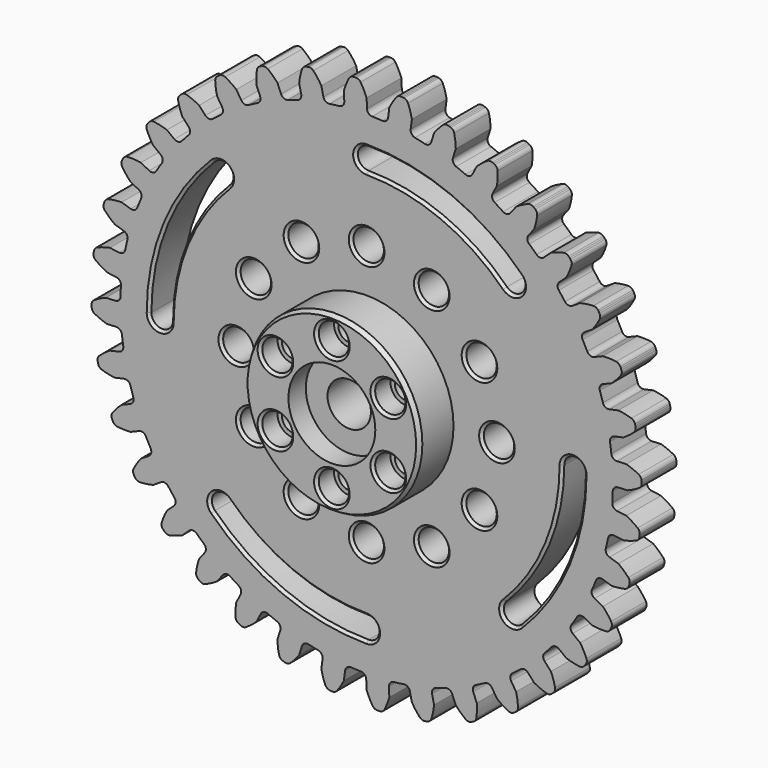
from build123d import *

# Parameters (mm, degrees)
F1_DEPTH       = 6.35
F2_R           = 2.2225
F3_DEPTH       = 25.4
F4_R           = 12.7
F5_DEPTH       = 6.35
F7_D           = 3.175
F7_CBORE_D     = 4.445
F7_CBORE_DEPTH = 3.175
F8_D           = 6.35
F8_CBORE_D     = 12.7
F8_CBORE_DEPTH = 3.175
F9_SIZE2       = 0.6599113577
F9_SIZE        = 0.381
F10_SIZE2      = 0.381
F10_SIZE       = 0.381


with BuildPart() as f1:
    # F0 (on Front) → F1 (new body)
    with BuildSketch(Plane.XZ):
        with BuildLine():
            ThreePointArc((-3.2606716013, 36.5816578877), (-3.4493856486, 36.0349930627), (-3.9606537478, 35.7646962753))
            ThreePointArc((-3.9606537478, 35.7646962753), (-4.6967674834, 35.6754909284), (-5.4308867943, 35.5711364227))
            ThreePointArc((-5.4308867943, 35.5711364227), (-5.9946918119, 35.6998971492), (-6.318462852, 36.1790920324))
            Line((-6.318462852, 36.1790920324), (-6.6159955691, 37.5211753898))
            ThreePointArc((-6.6159955691, 37.5211753898), (-7.1619458758, 38.3313229182), (-7.7880082615, 39.081287347))
            ThreePointArc((-7.7880082615, 39.081287347), (-8.1146145803, 39.2926127714), (-8.5025305694, 39.3217899538))
            Line((-8.5025305694, 39.3217899538), (-8.7093463733, 39.2853227475))
            Line((-8.7093463733, 39.2853227475), (-8.9121968543, 39.2309691249))
            ThreePointArc((-8.9121968543, 39.2309691249), (-9.2514373257, 39.0405852364), (-9.4581331923, 38.7110295639))
            ThreePointArc((-9.4581331923, 38.7110295639), (-9.7085897444, 37.7667455649), (-9.8610056184, 36.8017739816))
            Line((-9.8610056184, 36.8017739816), (-9.5634729013, 35.4596906243))
            ThreePointArc((-9.5634729013, 35.4596906243), (-9.6543926075, 34.8885610159), (-10.1109568509, 34.5335898704))
            ThreePointArc((-10.1109568509, 34.5335898704), (-10.8203970188, 34.3179149444), (-11.5252424382, 34.0876673376))
            ThreePointArc((-11.5252424382, 34.0876673376), (-12.1028410562, 34.1165681854), (-12.5049046048, 34.5322607706))
            Line((-12.5049046048, 34.5322607706), (-13.0309674607, 35.8022888519))
            ThreePointArc((-13.0309674607, 35.8022888519), (-13.7093041974, 36.5053251432), (-14.4560852451, 37.1351813348))
            ThreePointArc((-14.4560852451, 37.1351813348), (-14.8144259549, 37.286581659), (-15.201515193, 37.2479546698))
            Line((-15.201515193, 37.2479546698), (-15.3988565363, 37.1761282949))
            Line((-15.3988565363, 37.1761282949), (-15.5891868551, 37.0873758097))
            ThreePointArc((-15.5891868551, 37.0873758097), (-15.8902136862, 36.8409757905), (-16.0365426362, 36.4805344486))
            ThreePointArc((-16.0365426362, 36.4805344486), (-16.1192209948, 35.5071049215), (-16.1017557723, 34.5303266861))
            Line((-16.1017557723, 34.5303266861), (-15.5756929164, 33.2602986047))
            ThreePointArc((-15.5756929164, 33.2602986047), (-15.5660557323, 32.6820576972), (-15.9540436464, 32.2531978121))
            ThreePointArc((-15.9540436464, 32.2531978121), (-16.6152542662, 31.9176064805), (-17.2694094225, 31.5684617296))
            ThreePointArc((-17.2694094225, 31.5684617296), (-17.8432515992, 31.4966245612), (-18.311391159, 31.8361842394))
            Line((-18.311391159, 31.8361842394), (-19.05, 32.9955678842))
            ThreePointArc((-19.05, 32.9955678842), (-19.8401122483, 33.5701315363), (-20.6849213937, 34.060741629))
            ThreePointArc((-20.6849213937, 34.060741629), (-21.0641084934, 34.1476166309), (-21.4386094698, 34.0423591317))
            Line((-21.4386094698, 34.0423591317), (-21.6204802356, 33.9373559961))
            Line((-21.6204802356, 33.9373559961), (-21.7925073018, 33.8169013475))
            ThreePointArc((-21.7925073018, 33.8169013475), (-22.0461739447, 33.5219719377), (-22.127689847, 33.1415967542))
            ThreePointArc((-22.127689847, 33.1415967542), (-22.0400778721, 32.1685988626), (-21.853262225, 31.2096928874))
            Line((-21.853262225, 31.2096928874), (-21.114653384, 30.0503092426))
            ThreePointArc((-21.114653384, 30.0503092426), (-21.0047521305, 29.4825265932), (-21.3123748989, 28.9928086592))
            ThreePointArc((-21.3123748989, 28.9928086592), (-21.9052654205, 28.5474976948), (-22.4888541403, 28.0900643864))
            ThreePointArc((-22.4888541403, 28.0900643864), (-23.0415039716, 27.9196719377), (-23.5614953589, 28.17278136))
            Line((-23.5614953589, 28.17278136), (-24.4902079291, 29.1862932828))
            ThreePointArc((-24.4902079291, 29.1862932828), (-25.3680885281, 29.61492647), (-26.2852566728, 29.9513835244))
            ThreePointArc((-26.2852566728, 29.9513835244), (-26.6737687542, 29.9710935509), (-27.0243024464, 29.8024037375))
            Line((-27.0243024464, 29.8024037375), (-27.1851765834, 29.6674143085))
            Line((-27.1851765834, 29.6674143085), (-27.3336734418, 29.5189174501))
            ThreePointArc((-27.3336734418, 29.5189174501), (-27.5322723638, 29.1844199304), (-27.5464983989, 28.7956684128))
            ThreePointArc((-27.5464983989, 28.7956684128), (-27.291258136, 27.8526662053), (-26.9407683632, 26.9407683632))
            Line((-26.9407683632, 26.9407683632), (-26.012055793, 25.9272564403))
            ThreePointArc((-26.012055793, 25.9272564403), (-25.8052297641, 25.3871838375), (-26.0231404246, 24.8514876862))
            ThreePointArc((-26.0231404246, 24.8514876862), (-26.5296961696, 24.3099876374), (-27.024986405, 23.758164651))
            ThreePointArc((-27.024986405, 23.758164651), (-27.5396519053, 23.4943942104), (-28.095695445, 23.653362775))
            Line((-28.095695445, 23.653362775), (-29.1862932828, 24.4902079291))
            ThreePointArc((-29.1862932828, 24.4902079291), (-30.1252682748, 24.7598868487), (-31.0869277289, 24.9319677875))
            ThreePointArc((-31.0869277289, 24.9319677875), (-31.472960049, 24.8839139595), (-31.7888756681, 24.6569173866))
            Line((-31.7888756681, 24.6569173866), (-31.9238650971, 24.4960432496))
            Line((-31.9238650971, 24.4960432496), (-32.0443197457, 24.3240161833))
            ThreePointArc((-32.0443197457, 24.3240161833), (-32.1818166191, 23.9601140917), (-32.1283205362, 23.5747982581))
            ThreePointArc((-32.1283205362, 23.5747982581), (-31.7132073315, 22.6904443795), (-31.2096928874, 21.853262225))
            Line((-31.2096928874, 21.853262225), (-30.1190950495, 21.0164170709))
            ThreePointArc((-30.1190950495, 21.0164170709), (-29.8216285495, 20.5204643475), (-29.9432059969, 19.9550668353))
            ThreePointArc((-29.9432059969, 19.9550668353), (-30.3480355252, 19.333830907), (-30.7399781331, 18.704385105))
            ThreePointArc((-30.7399781331, 18.704385105), (-31.2010214516, 18.3552512038), (-31.7762220421, 18.4152487314))
            Line((-31.7762220421, 18.4152487314), (-32.9955678842, 19.05))
            ThreePointArc((-32.9955678842, 19.05), (-33.9671069891, 19.1525305947), (-34.9440382167, 19.1550068256))
            ThreePointArc((-34.9440382167, 19.1550068256), (-35.3158613788, 19.0406492343), (-35.5875599885, 18.7622430779))
            Line((-35.5875599885, 18.7622430779), (-35.6925631241, 18.5803723121))
            Line((-35.6925631241, 18.5803723121), (-35.7813156093, 18.3900419933))
            ThreePointArc((-35.7813156093, 18.3900419933), (-35.8535326612, 18.0077923106), (-35.7339399116, 17.6376197876))
            ThreePointArc((-35.7339399116, 17.6376197876), (-35.1715667699, 16.8387848831), (-34.5303266861, 16.1017557723))
            Line((-34.5303266861, 16.1017557723), (-33.310980844, 15.4670045037))
            ThreePointArc((-33.310980844, 15.4670045037), (-32.9319122418, 15.0302409322), (-32.953462407, 14.4523213765))
            ThreePointArc((-32.953462407, 14.4523213765), (-33.2442651782, 13.7702255079), (-33.5209511807, 13.0822822824))
            ThreePointArc((-33.5209511807, 13.0822822824), (-33.9143637496, 12.6583931776), (-34.4912442119, 12.6175966735))
            Line((-34.4912442119, 12.6175966735), (-35.8022888519, 13.0309674607))
            ThreePointArc((-35.8022888519, 13.0309674607), (-36.7768723457, 12.9632343902), (-37.7393917859, 12.7960306742))
            ThreePointArc((-37.7393917859, 12.7960306742), (-38.0857081313, 12.6188440172), (-38.3049343069, 12.2974875074))
            Line((-38.3049343069, 12.2974875074), (-38.3767606818, 12.1001461641))
            Line((-38.3767606818, 12.1001461641), (-38.4311143044, 11.8972956831))
            ThreePointArc((-38.4311143044, 11.8972956831), (-38.4358572562, 11.5083128726), (-38.2538016052, 11.164531165))
            ThreePointArc((-38.2538016052, 11.164531165), (-37.5612559497, 10.4754874289), (-36.8017739816, 9.8610056184))
            Line((-36.8017739816, 9.8610056184), (-35.4907293416, 9.4476348312))
            ThreePointArc((-35.4907293416, 9.4476348312), (-35.041576445, 9.0833312518), (-34.9624445371, 8.5104494458))
            ThreePointArc((-34.9624445371, 8.5104494458), (-35.1303846562, 7.7882187749), (-35.2834070892, 7.0626809326))
            ThreePointArc((-35.2834070892, 7.0626809326), (-35.5972352666, 6.5769162801), (-36.1582673798, 6.4365653256))
            Line((-36.1582673798, 6.4365653256), (-37.5211753898, 6.6159955691))
            ThreePointArc((-37.5211753898, 6.6159955691), (-38.4691910462, 6.3800568684), (-39.3880530326, 6.0482536059))
            ThreePointArc((-39.3880530326, 6.0482536059), (-39.6983399145, 5.81362161), (-39.8584325796, 5.4590790018))
            Line((-39.8584325796, 5.4590790018), (-39.8948997859, 5.2522631978))
            Line((-39.8948997859, 5.2522631978), (-39.9132030384, 5.043056064))
            ThreePointArc((-39.9132030384, 5.043056064), (-39.8503277779, 4.6591591714), (-39.6113408943, 4.3522139125))
            ThreePointArc((-39.6113408943, 4.3522139125), (-38.8096653743, 3.79389759), (-37.9550179973, 3.3206337987))
            Line((-37.9550179973, 3.3206337987), (-36.5921099874, 3.1412035552))
            ThreePointArc((-36.5921099874, 3.1412035552), (-36.0865200798, 2.8604291477), (-35.9091104818, 2.3099918152))
            ThreePointArc((-35.9091104818, 2.3099918152), (-35.9490851733, 1.5695709554), (-35.9737945275, 0.8284835965))
            ThreePointArc((-35.9737945275, 0.8284835965), (-36.198502803, 0.2956031095), (-36.7266398904, 0.0599621973))
            Line((-36.7266398904, 0.0599621973), (-38.1, 0))
            ThreePointArc((-38.1, 0), (-38.992642843, -0.3969754528), (-39.8399282193, -0.8832965877))
            ThreePointArc((-39.8399282193, -0.8832965877), (-40.1047577277, -1.1682447479), (-40.2008525477, -1.5452008569))
            Line((-40.2008525477, -1.5452008569), (-40.2008525477, -1.755207128))
            Line((-40.2008525477, -1.755207128), (-40.1825492952, -1.9644142618))
            ThreePointArc((-40.1825492952, -1.9644142618), (-40.0539662553, -2.3315607235), (-39.7653096346, -2.5923431574))
            ThreePointArc((-39.7653096346, -2.5923431574), (-38.8788627552, -3.0029679073), (-37.9550179973, -3.3206337987))
            Line((-37.9550179973, -3.3206337987), (-36.5816578877, -3.2606716013))
            ThreePointArc((-36.5816578877, -3.2606716013), (-36.0349930627, -3.4493856486), (-35.7646962753, -3.9606537478))
            ThreePointArc((-35.7646962753, -3.9606537478), (-35.6754909284, -4.6967674834), (-35.5711364227, -5.4308867943))
            ThreePointArc((-35.5711364227, -5.4308867943), (-35.6998971492, -5.9946918119), (-36.1790920324, -6.318462852))
            Line((-36.1790920324, -6.318462852), (-37.5211753898, -6.6159955691))
            ThreePointArc((-37.5211753898, -6.6159955691), (-38.3313229182, -7.1619458758), (-39.081287347, -7.7880082615))
            ThreePointArc((-39.081287347, -7.7880082615), (-39.2926127714, -8.1146145803), (-39.3217899538, -8.5025305694))
            Line((-39.3217899538, -8.5025305694), (-39.2853227475, -8.7093463733))
            Line((-39.2853227475, -8.7093463733), (-39.2309691249, -8.9121968543))
            ThreePointArc((-39.2309691249, -8.9121968543), (-39.0405852364, -9.2514373257), (-38.7110295639, -9.4581331923))
            ThreePointArc((-38.7110295639, -9.4581331923), (-37.7667455649, -9.7085897444), (-36.8017739816, -9.8610056184))
            Line((-36.8017739816, -9.8610056184), (-35.4596906243, -9.5634729013))
            ThreePointArc((-35.4596906243, -9.5634729013), (-34.8885610159, -9.6543926075), (-34.5335898704, -10.1109568509))
            ThreePointArc((-34.5335898704, -10.1109568509), (-34.3179149444, -10.8203970188), (-34.0876673376, -11.5252424382))
            ThreePointArc((-34.0876673376, -11.5252424382), (-34.1165681854, -12.1028410562), (-34.5322607706, -12.5049046048))
            Line((-34.5322607706, -12.5049046048), (-35.8022888519, -13.0309674607))
            ThreePointArc((-35.8022888519, -13.0309674607), (-36.5053251432, -13.7093041974), (-37.1351813348, -14.4560852451))
            ThreePointArc((-37.1351813348, -14.4560852451), (-37.286581659, -14.8144259549), (-37.2479546698, -15.201515193))
            Line((-37.2479546698, -15.201515193), (-37.1761282949, -15.3988565363))
            Line((-37.1761282949, -15.3988565363), (-37.0873758097, -15.5891868551))
            ThreePointArc((-37.0873758097, -15.5891868551), (-36.8409757905, -15.8902136862), (-36.4805344486, -16.0365426362))
            ThreePointArc((-36.4805344486, -16.0365426362), (-35.5071049215, -16.1192209948), (-34.5303266861, -16.1017557723))
            Line((-34.5303266861, -16.1017557723), (-33.2602986047, -15.5756929164))
            ThreePointArc((-33.2602986047, -15.5756929164), (-32.6820576972, -15.5660557323), (-32.2531978121, -15.9540436464))
            ThreePointArc((-32.2531978121, -15.9540436464), (-31.9176064805, -16.6152542662), (-31.5684617296, -17.2694094225))
            ThreePointArc((-31.5684617296, -17.2694094225), (-31.4966245612, -17.8432515992), (-31.8361842394, -18.311391159))
            Line((-31.8361842394, -18.311391159), (-32.9955678842, -19.05))
            ThreePointArc((-32.9955678842, -19.05), (-33.5701315363, -19.8401122483), (-34.060741629, -20.6849213937))
            ThreePointArc((-34.060741629, -20.6849213937), (-34.1476166309, -21.0641084934), (-34.0423591317, -21.4386094698))
            Line((-34.0423591317, -21.4386094698), (-33.9373559961, -21.6204802356))
            Line((-33.9373559961, -21.6204802356), (-33.8169013475, -21.7925073018))
            ThreePointArc((-33.8169013475, -21.7925073018), (-33.5219719377, -22.0461739447), (-33.1415967542, -22.127689847))
            ThreePointArc((-33.1415967542, -22.127689847), (-32.1685988626, -22.0400778721), (-31.2096928874, -21.853262225))
            Line((-31.2096928874, -21.853262225), (-30.0503092426, -21.114653384))
            ThreePointArc((-30.0503092426, -21.114653384), (-29.4825265932, -21.0047521305), (-28.9928086592, -21.3123748989))
            ThreePointArc((-28.9928086592, -21.3123748989), (-28.5474976948, -21.9052654205), (-28.0900643864, -22.4888541403))
            ThreePointArc((-28.0900643864, -22.4888541403), (-27.9196719377, -23.0415039716), (-28.17278136, -23.5614953589))
            Line((-28.17278136, -23.5614953589), (-29.1862932828, -24.4902079291))
            ThreePointArc((-29.1862932828, -24.4902079291), (-29.61492647, -25.3680885281), (-29.9513835244, -26.2852566728))
            ThreePointArc((-29.9513835244, -26.2852566728), (-29.9710935509, -26.6737687542), (-29.8024037375, -27.0243024464))
            Line((-29.8024037375, -27.0243024464), (-29.6674143085, -27.1851765834))
            Line((-29.6674143085, -27.1851765834), (-29.5189174501, -27.3336734418))
            ThreePointArc((-29.5189174501, -27.3336734418), (-29.1844199304, -27.5322723638), (-28.7956684128, -27.5464983989))
            ThreePointArc((-28.7956684128, -27.5464983989), (-27.8526662053, -27.291258136), (-26.9407683632, -26.9407683632))
            Line((-26.9407683632, -26.9407683632), (-25.9272564403, -26.012055793))
            ThreePointArc((-25.9272564403, -26.012055793), (-25.3871838375, -25.8052297641), (-24.8514876862, -26.0231404246))
            ThreePointArc((-24.8514876862, -26.0231404246), (-24.3099876374, -26.5296961696), (-23.758164651, -27.024986405))
            ThreePointArc((-23.758164651, -27.024986405), (-23.4943942104, -27.5396519053), (-23.653362775, -28.095695445))
            Line((-23.653362775, -28.095695445), (-24.4902079291, -29.1862932828))
            ThreePointArc((-24.4902079291, -29.1862932828), (-24.7598868487, -30.1252682748), (-24.9319677875, -31.0869277289))
            ThreePointArc((-24.9319677875, -31.0869277289), (-24.8839139595, -31.472960049), (-24.6569173866, -31.7888756681))
            Line((-24.6569173866, -31.7888756681), (-24.4960432496, -31.9238650971))
            Line((-24.4960432496, -31.9238650971), (-24.3240161833, -32.0443197457))
            ThreePointArc((-24.3240161833, -32.0443197457), (-23.9601140917, -32.1818166191), (-23.5747982581, -32.1283205362))
            ThreePointArc((-23.5747982581, -32.1283205362), (-22.6904443795, -31.7132073315), (-21.853262225, -31.2096928874))
            Line((-21.853262225, -31.2096928874), (-21.0164170709, -30.1190950495))
            ThreePointArc((-21.0164170709, -30.1190950495), (-20.5204643475, -29.8216285495), (-19.9550668353, -29.9432059969))
            ThreePointArc((-19.9550668353, -29.9432059969), (-19.333830907, -30.3480355252), (-18.704385105, -30.7399781331))
            ThreePointArc((-18.704385105, -30.7399781331), (-18.3552512038, -31.2010214516), (-18.4152487314, -31.7762220421))
            Line((-18.4152487314, -31.7762220421), (-19.05, -32.9955678842))
            ThreePointArc((-19.05, -32.9955678842), (-19.1525305947, -33.9671069891), (-19.1550068256, -34.9440382167))
            ThreePointArc((-19.1550068256, -34.9440382167), (-19.0406492343, -35.3158613788), (-18.7622430779, -35.5875599885))
            Line((-18.7622430779, -35.5875599885), (-18.5803723121, -35.6925631241))
            Line((-18.5803723121, -35.6925631241), (-18.3900419933, -35.7813156093))
            ThreePointArc((-18.3900419933, -35.7813156093), (-18.0077923106, -35.8535326612), (-17.6376197876, -35.7339399116))
            ThreePointArc((-17.6376197876, -35.7339399116), (-16.8387848831, -35.1715667699), (-16.1017557723, -34.5303266861))
            Line((-16.1017557723, -34.5303266861), (-15.4670045037, -33.310980844))
            ThreePointArc((-15.4670045037, -33.310980844), (-15.0302409322, -32.9319122418), (-14.4523213765, -32.953462407))
            ThreePointArc((-14.4523213765, -32.953462407), (-13.7702255079, -33.2442651782), (-13.0822822824, -33.5209511807))
            ThreePointArc((-13.0822822824, -33.5209511807), (-12.6583931776, -33.9143637496), (-12.6175966735, -34.4912442119))
            Line((-12.6175966735, -34.4912442119), (-13.0309674607, -35.8022888519))
            ThreePointArc((-13.0309674607, -35.8022888519), (-12.9632343902, -36.7768723457), (-12.7960306742, -37.7393917859))
            ThreePointArc((-12.7960306742, -37.7393917859), (-12.6188440172, -38.0857081313), (-12.2974875074, -38.3049343069))
            Line((-12.2974875074, -38.3049343069), (-12.1001461641, -38.3767606818))
            Line((-12.1001461641, -38.3767606818), (-11.8972956831, -38.4311143044))
            ThreePointArc((-11.8972956831, -38.4311143044), (-11.5083128726, -38.4358572562), (-11.164531165, -38.2538016052))
            ThreePointArc((-11.164531165, -38.2538016052), (-10.4754874289, -37.5612559497), (-9.8610056184, -36.8017739816))
            Line((-9.8610056184, -36.8017739816), (-9.4476348312, -35.4907293416))
            ThreePointArc((-9.4476348312, -35.4907293416), (-9.0833312518, -35.041576445), (-8.5104494458, -34.9624445371))
            ThreePointArc((-8.5104494458, -34.9624445371), (-7.7882187749, -35.1303846562), (-7.0626809326, -35.2834070892))
            ThreePointArc((-7.0626809326, -35.2834070892), (-6.5769162801, -35.5972352666), (-6.4365653256, -36.1582673798))
            Line((-6.4365653256, -36.1582673798), (-6.6159955691, -37.5211753898))
            ThreePointArc((-6.6159955691, -37.5211753898), (-6.3800568684, -38.4691910462), (-6.0482536059, -39.3880530326))
            ThreePointArc((-6.0482536059, -39.3880530326), (-5.81362161, -39.6983399145), (-5.4590790018, -39.8584325796))
            Line((-5.4590790018, -39.8584325796), (-5.2522631978, -39.8948997859))
            Line((-5.2522631978, -39.8948997859), (-5.043056064, -39.9132030384))
            ThreePointArc((-5.043056064, -39.9132030384), (-4.6591591714, -39.8503277779), (-4.3522139125, -39.6113408943))
            ThreePointArc((-4.3522139125, -39.6113408943), (-3.79389759, -38.8096653743), (-3.3206337987, -37.9550179973))
            Line((-3.3206337987, -37.9550179973), (-3.1412035552, -36.5921099874))
            ThreePointArc((-3.1412035552, -36.5921099874), (-2.8604291477, -36.0865200798), (-2.3099918152, -35.9091104818))
            ThreePointArc((-2.3099918152, -35.9091104818), (-1.5695709554, -35.9490851733), (-0.8284835965, -35.9737945275))
            ThreePointArc((-0.8284835965, -35.9737945275), (-0.2956031095, -36.198502803), (-0.0599621973, -36.7266398904))
            Line((-0.0599621973, -36.7266398904), (0, -38.1))
            ThreePointArc((0, -38.1), (0.3969754528, -38.992642843), (0.8832965877, -39.8399282193))
            ThreePointArc((0.8832965877, -39.8399282193), (1.1682447479, -40.1047577277), (1.5452008569, -40.2008525477))
            Line((1.5452008569, -40.2008525477), (1.755207128, -40.2008525477))
            Line((1.755207128, -40.2008525477), (1.9644142618, -40.1825492952))
            ThreePointArc((1.9644142618, -40.1825492952), (2.3315607235, -40.0539662553), (2.5923431574, -39.7653096346))
            ThreePointArc((2.5923431574, -39.7653096346), (3.0029679073, -38.8788627552), (3.3206337987, -37.9550179973))
            Line((3.3206337987, -37.9550179973), (3.2606716013, -36.5816578877))
            ThreePointArc((3.2606716013, -36.5816578877), (3.4493856486, -36.0349930627), (3.9606537478, -35.7646962753))
            ThreePointArc((3.9606537478, -35.7646962753), (4.6967674834, -35.6754909284), (5.4308867943, -35.5711364227))
            ThreePointArc((5.4308867943, -35.5711364227), (5.9946918119, -35.6998971492), (6.318462852, -36.1790920324))
            Line((6.318462852, -36.1790920324), (6.6159955691, -37.5211753898))
            ThreePointArc((6.6159955691, -37.5211753898), (7.1619458758, -38.3313229182), (7.7880082615, -39.081287347))
            ThreePointArc((7.7880082615, -39.081287347), (8.1146145803, -39.2926127714), (8.5025305694, -39.3217899538))
            Line((8.5025305694, -39.3217899538), (8.7093463733, -39.2853227475))
            Line((8.7093463733, -39.2853227475), (8.9121968543, -39.2309691249))
            ThreePointArc((8.9121968543, -39.2309691249), (9.2514373257, -39.0405852364), (9.4581331923, -38.7110295639))
            ThreePointArc((9.4581331923, -38.7110295639), (9.7085897444, -37.7667455649), (9.8610056184, -36.8017739816))
            Line((9.8610056184, -36.8017739816), (9.5634729013, -35.4596906243))
            ThreePointArc((9.5634729013, -35.4596906243), (9.6543926075, -34.8885610159), (10.1109568509, -34.5335898704))
            ThreePointArc((10.1109568509, -34.5335898704), (10.8203970188, -34.3179149444), (11.5252424382, -34.0876673376))
            ThreePointArc((11.5252424382, -34.0876673376), (12.1028410562, -34.1165681854), (12.5049046048, -34.5322607706))
            Line((12.5049046048, -34.5322607706), (13.0309674607, -35.8022888519))
            ThreePointArc((13.0309674607, -35.8022888519), (13.7093041974, -36.5053251432), (14.4560852451, -37.1351813348))
            ThreePointArc((14.4560852451, -37.1351813348), (14.8144259549, -37.286581659), (15.201515193, -37.2479546698))
            Line((15.201515193, -37.2479546698), (15.3988565363, -37.1761282949))
            Line((15.3988565363, -37.1761282949), (15.5891868551, -37.0873758097))
            ThreePointArc((15.5891868551, -37.0873758097), (15.8902136862, -36.8409757905), (16.0365426362, -36.4805344486))
            ThreePointArc((16.0365426362, -36.4805344486), (16.1192209948, -35.5071049215), (16.1017557723, -34.5303266861))
            Line((16.1017557723, -34.5303266861), (15.5756929164, -33.2602986047))
            ThreePointArc((15.5756929164, -33.2602986047), (15.5660557323, -32.6820576972), (15.9540436464, -32.2531978121))
            ThreePointArc((15.9540436464, -32.2531978121), (16.6152542662, -31.9176064805), (17.2694094225, -31.5684617296))
            ThreePointArc((17.2694094225, -31.5684617296), (17.8432515992, -31.4966245612), (18.311391159, -31.8361842394))
            Line((18.311391159, -31.8361842394), (19.05, -32.9955678842))
            ThreePointArc((19.05, -32.9955678842), (19.8401122483, -33.5701315363), (20.6849213937, -34.060741629))
            ThreePointArc((20.6849213937, -34.060741629), (21.0641084934, -34.1476166309), (21.4386094698, -34.0423591317))
            Line((21.4386094698, -34.0423591317), (21.6204802356, -33.9373559961))
            Line((21.6204802356, -33.9373559961), (21.7925073018, -33.8169013475))
            ThreePointArc((21.7925073018, -33.8169013475), (22.0461739447, -33.5219719377), (22.127689847, -33.1415967542))
            ThreePointArc((22.127689847, -33.1415967542), (22.0400778721, -32.1685988626), (21.853262225, -31.2096928874))
            Line((21.853262225, -31.2096928874), (21.114653384, -30.0503092426))
            ThreePointArc((21.114653384, -30.0503092426), (21.0047521305, -29.4825265932), (21.3123748989, -28.9928086592))
            ThreePointArc((21.3123748989, -28.9928086592), (21.9052654205, -28.5474976948), (22.4888541403, -28.0900643864))
            ThreePointArc((22.4888541403, -28.0900643864), (23.0415039716, -27.9196719377), (23.5614953589, -28.17278136))
            Line((23.5614953589, -28.17278136), (24.4902079291, -29.1862932828))
            ThreePointArc((24.4902079291, -29.1862932828), (25.3680885281, -29.61492647), (26.2852566728, -29.9513835244))
            ThreePointArc((26.2852566728, -29.9513835244), (26.6737687542, -29.9710935509), (27.0243024464, -29.8024037375))
            Line((27.0243024464, -29.8024037375), (27.1851765834, -29.6674143085))
            Line((27.1851765834, -29.6674143085), (27.3336734418, -29.5189174501))
            ThreePointArc((27.3336734418, -29.5189174501), (27.5322723638, -29.1844199304), (27.5464983989, -28.7956684128))
            ThreePointArc((27.5464983989, -28.7956684128), (27.291258136, -27.8526662053), (26.9407683632, -26.9407683632))
            Line((26.9407683632, -26.9407683632), (26.012055793, -25.9272564403))
            ThreePointArc((26.012055793, -25.9272564403), (25.8052297641, -25.3871838375), (26.0231404246, -24.8514876862))
            ThreePointArc((26.0231404246, -24.8514876862), (26.5296961696, -24.3099876374), (27.024986405, -23.758164651))
            ThreePointArc((27.024986405, -23.758164651), (27.5396519053, -23.4943942104), (28.095695445, -23.653362775))
            Line((28.095695445, -23.653362775), (29.1862932828, -24.4902079291))
            ThreePointArc((29.1862932828, -24.4902079291), (30.1252682748, -24.7598868487), (31.0869277289, -24.9319677875))
            ThreePointArc((31.0869277289, -24.9319677875), (31.472960049, -24.8839139595), (31.7888756681, -24.6569173866))
            Line((31.7888756681, -24.6569173866), (31.9238650971, -24.4960432496))
            Line((31.9238650971, -24.4960432496), (32.0443197457, -24.3240161833))
            ThreePointArc((32.0443197457, -24.3240161833), (32.1818166191, -23.9601140917), (32.1283205362, -23.5747982581))
            ThreePointArc((32.1283205362, -23.5747982581), (31.7132073315, -22.6904443795), (31.2096928874, -21.853262225))
            Line((31.2096928874, -21.853262225), (30.1190950495, -21.0164170709))
            ThreePointArc((30.1190950495, -21.0164170709), (29.8216285495, -20.5204643475), (29.9432059969, -19.9550668353))
            ThreePointArc((29.9432059969, -19.9550668353), (30.3480355252, -19.333830907), (30.7399781331, -18.704385105))
            ThreePointArc((30.7399781331, -18.704385105), (31.2010214516, -18.3552512038), (31.7762220421, -18.4152487314))
            Line((31.7762220421, -18.4152487314), (32.9955678842, -19.05))
            ThreePointArc((32.9955678842, -19.05), (33.9671069891, -19.1525305947), (34.9440382167, -19.1550068256))
            ThreePointArc((34.9440382167, -19.1550068256), (35.3158613788, -19.0406492343), (35.5875599885, -18.7622430779))
            Line((35.5875599885, -18.7622430779), (35.6925631241, -18.5803723121))
            Line((35.6925631241, -18.5803723121), (35.7813156093, -18.3900419933))
            ThreePointArc((35.7813156093, -18.3900419933), (35.8535326612, -18.0077923106), (35.7339399116, -17.6376197876))
            ThreePointArc((35.7339399116, -17.6376197876), (35.1715667699, -16.8387848831), (34.5303266861, -16.1017557723))
            Line((34.5303266861, -16.1017557723), (33.310980844, -15.4670045037))
            ThreePointArc((33.310980844, -15.4670045037), (32.9319122418, -15.0302409322), (32.953462407, -14.4523213765))
            ThreePointArc((32.953462407, -14.4523213765), (33.2442651782, -13.7702255079), (33.5209511807, -13.0822822824))
            ThreePointArc((33.5209511807, -13.0822822824), (33.9143637496, -12.6583931776), (34.4912442119, -12.6175966735))
            Line((34.4912442119, -12.6175966735), (35.8022888519, -13.0309674607))
            ThreePointArc((35.8022888519, -13.0309674607), (36.7768723457, -12.9632343902), (37.7393917859, -12.7960306742))
            ThreePointArc((37.7393917859, -12.7960306742), (38.0857081313, -12.6188440172), (38.3049343069, -12.2974875074))
            Line((38.3049343069, -12.2974875074), (38.3767606818, -12.1001461641))
            Line((38.3767606818, -12.1001461641), (38.4311143044, -11.8972956831))
            ThreePointArc((38.4311143044, -11.8972956831), (38.4358572562, -11.5083128726), (38.2538016052, -11.164531165))
            ThreePointArc((38.2538016052, -11.164531165), (37.5612559497, -10.4754874289), (36.8017739816, -9.8610056184))
            Line((36.8017739816, -9.8610056184), (35.4907293416, -9.4476348312))
            ThreePointArc((35.4907293416, -9.4476348312), (35.041576445, -9.0833312518), (34.9624445371, -8.5104494458))
            ThreePointArc((34.9624445371, -8.5104494458), (35.1303846562, -7.7882187749), (35.2834070892, -7.0626809326))
            ThreePointArc((35.2834070892, -7.0626809326), (35.5972352666, -6.5769162801), (36.1582673798, -6.4365653256))
            Line((36.1582673798, -6.4365653256), (37.5211753898, -6.6159955691))
            ThreePointArc((37.5211753898, -6.6159955691), (38.4691910462, -6.3800568684), (39.3880530326, -6.0482536059))
            ThreePointArc((39.3880530326, -6.0482536059), (39.6983399145, -5.81362161), (39.8584325796, -5.4590790018))
            Line((39.8584325796, -5.4590790018), (39.8948997859, -5.2522631978))
            Line((39.8948997859, -5.2522631978), (39.9132030384, -5.043056064))
            ThreePointArc((39.9132030384, -5.043056064), (39.8503277779, -4.6591591714), (39.6113408943, -4.3522139125))
            ThreePointArc((39.6113408943, -4.3522139125), (38.8096653743, -3.79389759), (37.9550179973, -3.3206337987))
            Line((37.9550179973, -3.3206337987), (36.5921099874, -3.1412035552))
            ThreePointArc((36.5921099874, -3.1412035552), (36.0865200798, -2.8604291477), (35.9091104818, -2.3099918152))
            ThreePointArc((35.9091104818, -2.3099918152), (35.9490851733, -1.5695709554), (35.9737945275, -0.8284835965))
            ThreePointArc((35.9737945275, -0.8284835965), (36.198502803, -0.2956031095), (36.7266398904, -0.0599621973))
            Line((36.7266398904, -0.0599621973), (38.1, 0))
            ThreePointArc((38.1, 0), (38.992642843, 0.3969754528), (39.8399282193, 0.8832965877))
            ThreePointArc((39.8399282193, 0.8832965877), (40.1047577277, 1.1682447479), (40.2008525477, 1.5452008569))
            Line((40.2008525477, 1.5452008569), (40.2008525477, 1.755207128))
            Line((40.2008525477, 1.755207128), (40.1825492952, 1.9644142618))
            ThreePointArc((40.1825492952, 1.9644142618), (40.0539662553, 2.3315607235), (39.7653096346, 2.5923431574))
            ThreePointArc((39.7653096346, 2.5923431574), (38.8788627552, 3.0029679073), (37.9550179973, 3.3206337987))
            Line((37.9550179973, 3.3206337987), (36.5816578877, 3.2606716013))
            ThreePointArc((36.5816578877, 3.2606716013), (36.0349930627, 3.4493856486), (35.7646962753, 3.9606537478))
            ThreePointArc((35.7646962753, 3.9606537478), (35.6754909284, 4.6967674834), (35.5711364227, 5.4308867943))
            ThreePointArc((35.5711364227, 5.4308867943), (35.6998971492, 5.9946918119), (36.1790920324, 6.318462852))
            Line((36.1790920324, 6.318462852), (37.5211753898, 6.6159955691))
            ThreePointArc((37.5211753898, 6.6159955691), (38.3313229182, 7.1619458758), (39.081287347, 7.7880082615))
            ThreePointArc((39.081287347, 7.7880082615), (39.2926127714, 8.1146145803), (39.3217899538, 8.5025305694))
            Line((39.3217899538, 8.5025305694), (39.2853227475, 8.7093463733))
            Line((39.2853227475, 8.7093463733), (39.2309691249, 8.9121968543))
            ThreePointArc((39.2309691249, 8.9121968543), (39.0405852364, 9.2514373257), (38.7110295639, 9.4581331923))
            ThreePointArc((38.7110295639, 9.4581331923), (37.7667455649, 9.7085897444), (36.8017739816, 9.8610056184))
            Line((36.8017739816, 9.8610056184), (35.4596906243, 9.5634729013))
            ThreePointArc((35.4596906243, 9.5634729013), (34.8885610159, 9.6543926075), (34.5335898704, 10.1109568509))
            ThreePointArc((34.5335898704, 10.1109568509), (34.3179149444, 10.8203970188), (34.0876673376, 11.5252424382))
            ThreePointArc((34.0876673376, 11.5252424382), (34.1165681854, 12.1028410562), (34.5322607706, 12.5049046048))
            Line((34.5322607706, 12.5049046048), (35.8022888519, 13.0309674607))
            ThreePointArc((35.8022888519, 13.0309674607), (36.5053251432, 13.7093041974), (37.1351813348, 14.4560852451))
            ThreePointArc((37.1351813348, 14.4560852451), (37.286581659, 14.8144259549), (37.2479546698, 15.201515193))
            Line((37.2479546698, 15.201515193), (37.1761282949, 15.3988565363))
            Line((37.1761282949, 15.3988565363), (37.0873758097, 15.5891868551))
            ThreePointArc((37.0873758097, 15.5891868551), (36.8409757905, 15.8902136862), (36.4805344486, 16.0365426362))
            ThreePointArc((36.4805344486, 16.0365426362), (35.5071049215, 16.1192209948), (34.5303266861, 16.1017557723))
            Line((34.5303266861, 16.1017557723), (33.2602986047, 15.5756929164))
            ThreePointArc((33.2602986047, 15.5756929164), (32.6820576972, 15.5660557323), (32.2531978121, 15.9540436464))
            ThreePointArc((32.2531978121, 15.9540436464), (31.9176064805, 16.6152542662), (31.5684617296, 17.2694094225))
            ThreePointArc((31.5684617296, 17.2694094225), (31.4966245612, 17.8432515992), (31.8361842394, 18.311391159))
            Line((31.8361842394, 18.311391159), (32.9955678842, 19.05))
            ThreePointArc((32.9955678842, 19.05), (33.5701315363, 19.8401122483), (34.060741629, 20.6849213937))
            ThreePointArc((34.060741629, 20.6849213937), (34.1476166309, 21.0641084934), (34.0423591317, 21.4386094698))
            Line((34.0423591317, 21.4386094698), (33.9373559961, 21.6204802356))
            Line((33.9373559961, 21.6204802356), (33.8169013475, 21.7925073018))
            ThreePointArc((33.8169013475, 21.7925073018), (33.5219719377, 22.0461739447), (33.1415967542, 22.127689847))
            ThreePointArc((33.1415967542, 22.127689847), (32.1685988626, 22.0400778721), (31.2096928874, 21.853262225))
            Line((31.2096928874, 21.853262225), (30.0503092426, 21.114653384))
            ThreePointArc((30.0503092426, 21.114653384), (29.4825265932, 21.0047521305), (28.9928086592, 21.3123748989))
            ThreePointArc((28.9928086592, 21.3123748989), (28.5474976948, 21.9052654205), (28.0900643864, 22.4888541403))
            ThreePointArc((28.0900643864, 22.4888541403), (27.9196719377, 23.0415039716), (28.17278136, 23.5614953589))
            Line((28.17278136, 23.5614953589), (29.1862932828, 24.4902079291))
            ThreePointArc((29.1862932828, 24.4902079291), (29.61492647, 25.3680885281), (29.9513835244, 26.2852566728))
            ThreePointArc((29.9513835244, 26.2852566728), (29.9710935509, 26.6737687542), (29.8024037375, 27.0243024464))
            Line((29.8024037375, 27.0243024464), (29.6674143085, 27.1851765834))
            Line((29.6674143085, 27.1851765834), (29.5189174501, 27.3336734418))
            ThreePointArc((29.5189174501, 27.3336734418), (29.1844199304, 27.5322723638), (28.7956684128, 27.5464983989))
            ThreePointArc((28.7956684128, 27.5464983989), (27.8526662053, 27.291258136), (26.9407683632, 26.9407683632))
            Line((26.9407683632, 26.9407683632), (25.9272564403, 26.012055793))
            ThreePointArc((25.9272564403, 26.012055793), (25.3871838375, 25.8052297641), (24.8514876862, 26.0231404246))
            ThreePointArc((24.8514876862, 26.0231404246), (24.3099876374, 26.5296961696), (23.758164651, 27.024986405))
            ThreePointArc((23.758164651, 27.024986405), (23.4943942104, 27.5396519053), (23.653362775, 28.095695445))
            Line((23.653362775, 28.095695445), (24.4902079291, 29.1862932828))
            ThreePointArc((24.4902079291, 29.1862932828), (24.7598868487, 30.1252682748), (24.9319677875, 31.0869277289))
            ThreePointArc((24.9319677875, 31.0869277289), (24.8839139595, 31.472960049), (24.6569173866, 31.7888756681))
            Line((24.6569173866, 31.7888756681), (24.4960432496, 31.9238650971))
            Line((24.4960432496, 31.9238650971), (24.3240161833, 32.0443197457))
            ThreePointArc((24.3240161833, 32.0443197457), (23.9601140917, 32.1818166191), (23.5747982581, 32.1283205362))
            ThreePointArc((23.5747982581, 32.1283205362), (22.6904443795, 31.7132073315), (21.853262225, 31.2096928874))
            Line((21.853262225, 31.2096928874), (21.0164170709, 30.1190950495))
            ThreePointArc((21.0164170709, 30.1190950495), (20.5204643475, 29.8216285495), (19.9550668353, 29.9432059969))
            ThreePointArc((19.9550668353, 29.9432059969), (19.333830907, 30.3480355252), (18.704385105, 30.7399781331))
            ThreePointArc((18.704385105, 30.7399781331), (18.3552512038, 31.2010214516), (18.4152487314, 31.7762220421))
            Line((18.4152487314, 31.7762220421), (19.05, 32.9955678842))
            ThreePointArc((19.05, 32.9955678842), (19.1525305947, 33.9671069891), (19.1550068256, 34.9440382167))
            ThreePointArc((19.1550068256, 34.9440382167), (19.0406492343, 35.3158613788), (18.7622430779, 35.5875599885))
            Line((18.7622430779, 35.5875599885), (18.5803723121, 35.6925631241))
            Line((18.5803723121, 35.6925631241), (18.3900419933, 35.7813156093))
            ThreePointArc((18.3900419933, 35.7813156093), (18.0077923106, 35.8535326612), (17.6376197876, 35.7339399116))
            ThreePointArc((17.6376197876, 35.7339399116), (16.8387848831, 35.1715667699), (16.1017557723, 34.5303266861))
            Line((16.1017557723, 34.5303266861), (15.4670045037, 33.310980844))
            ThreePointArc((15.4670045037, 33.310980844), (15.0302409322, 32.9319122418), (14.4523213765, 32.953462407))
            ThreePointArc((14.4523213765, 32.953462407), (13.7702255079, 33.2442651782), (13.0822822824, 33.5209511807))
            ThreePointArc((13.0822822824, 33.5209511807), (12.6583931776, 33.9143637496), (12.6175966735, 34.4912442119))
            Line((12.6175966735, 34.4912442119), (13.0309674607, 35.8022888519))
            ThreePointArc((13.0309674607, 35.8022888519), (12.9632343902, 36.7768723457), (12.7960306742, 37.7393917859))
            ThreePointArc((12.7960306742, 37.7393917859), (12.6188440172, 38.0857081313), (12.2974875074, 38.3049343069))
            Line((12.2974875074, 38.3049343069), (12.1001461641, 38.3767606818))
            Line((12.1001461641, 38.3767606818), (11.8972956831, 38.4311143044))
            ThreePointArc((11.8972956831, 38.4311143044), (11.5083128726, 38.4358572562), (11.164531165, 38.2538016052))
            ThreePointArc((11.164531165, 38.2538016052), (10.4754874289, 37.5612559497), (9.8610056184, 36.8017739816))
            Line((9.8610056184, 36.8017739816), (9.4476348312, 35.4907293416))
            ThreePointArc((9.4476348312, 35.4907293416), (9.0833312518, 35.041576445), (8.5104494458, 34.9624445371))
            ThreePointArc((8.5104494458, 34.9624445371), (7.7882187749, 35.1303846562), (7.0626809326, 35.2834070892))
            ThreePointArc((7.0626809326, 35.2834070892), (6.5769162801, 35.5972352666), (6.4365653256, 36.1582673798))
            Line((6.4365653256, 36.1582673798), (6.6159955691, 37.5211753898))
            ThreePointArc((6.6159955691, 37.5211753898), (6.3800568684, 38.4691910462), (6.0482536059, 39.3880530326))
            ThreePointArc((6.0482536059, 39.3880530326), (5.81362161, 39.6983399145), (5.4590790018, 39.8584325796))
            Line((5.4590790018, 39.8584325796), (5.2522631978, 39.8948997859))
            Line((5.2522631978, 39.8948997859), (5.043056064, 39.9132030384))
            ThreePointArc((5.043056064, 39.9132030384), (4.6591591714, 39.8503277779), (4.3522139125, 39.6113408943))
            ThreePointArc((4.3522139125, 39.6113408943), (3.79389759, 38.8096653743), (3.3206337987, 37.9550179973))
            Line((3.3206337987, 37.9550179973), (3.1412035552, 36.5921099874))
            ThreePointArc((3.1412035552, 36.5921099874), (2.8604291477, 36.0865200798), (2.3099918152, 35.9091104818))
            ThreePointArc((2.3099918152, 35.9091104818), (1.5695709554, 35.9490851733), (0.8284835965, 35.9737945275))
            ThreePointArc((0.8284835965, 35.9737945275), (0.2956031095, 36.198502803), (0.0599621973, 36.7266398904))
            Line((0.0599621973, 36.7266398904), (0, 38.1))
            ThreePointArc((0, 38.1), (-0.3969754528, 38.992642843), (-0.8832965877, 39.8399282193))
            ThreePointArc((-0.8832965877, 39.8399282193), (-1.1682447479, 40.1047577277), (-1.5452008569, 40.2008525477))
            Line((-1.5452008569, 40.2008525477), (-1.755207128, 40.2008525477))
            Line((-1.755207128, 40.2008525477), (-1.9644142618, 40.1825492952))
            ThreePointArc((-1.9644142618, 40.1825492952), (-2.3315607235, 40.0539662553), (-2.5923431574, 39.7653096346))
            ThreePointArc((-2.5923431574, 39.7653096346), (-3.0029679073, 38.8788627552), (-3.3206337987, 37.9550179973))
            Line((-3.3206337987, 37.9550179973), (-3.2606716013, 36.5816578877))
        make_face()
    extrude(amount=F1_DEPTH)

    # F2 (on face) → F3 (cut)
    with BuildSketch(Plane.XZ.offset(6.35)):
        with BuildLine():
            ThreePointArc((22.4596205588, 22.4596205588), (12.1550590572, 29.3449084273), (0, 31.7627))
            ThreePointArc((0, 31.7627), (-1.5875, 30.1752), (0, 28.5877))
            ThreePointArc((0, 28.5877), (10.9400391594, 26.4115909116), (20.2145565285, 20.2145565285))
            ThreePointArc((20.2145565285, 20.2145565285), (22.4596205588, 20.2145565285), (22.4596205588, 22.4596205588))
        make_face()
        with BuildLine():
            ThreePointArc((-28.5877, 0), (-26.4115909116, 10.9400391594), (-20.2145565285, 20.2145565285))
            ThreePointArc((-20.2145565285, 20.2145565285), (-20.2145565285, 22.4596205588), (-22.4596205588, 22.4596205588))
            ThreePointArc((-22.4596205588, 22.4596205588), (-29.3449084273, 12.1550590572), (-31.7627, 0))
            ThreePointArc((-31.7627, 0), (-30.1752, -1.5875), (-28.5877, 0))
        make_face()
        with BuildLine():
            ThreePointArc((0, -28.5877), (-10.9400391594, -26.4115909116), (-20.2145565285, -20.2145565285))
            ThreePointArc((-20.2145565285, -20.2145565285), (-22.4596205588, -20.2145565285), (-22.4596205588, -22.4596205588))
            ThreePointArc((-22.4596205588, -22.4596205588), (-12.1550590572, -29.3449084273), (0, -31.7627))
            ThreePointArc((0, -31.7627), (1.5875, -30.1752), (0, -28.5877))
        make_face()
        with BuildLine():
            ThreePointArc((28.5877, 0), (26.4115909116, -10.9400391594), (20.2145565285, -20.2145565285))
            ThreePointArc((20.2145565285, -20.2145565285), (20.2145565285, -22.4596205588), (22.4596205588, -22.4596205588))
            ThreePointArc((22.4596205588, -22.4596205588), (29.3449084273, -12.1550590572), (31.7627, 0))
            ThreePointArc((31.7627, 0), (30.1752, 1.5875), (28.5877, 0))
        make_face()
        with Locations((0, 19.05)):
            Circle(F2_R)
        with Locations((-9.525, 16.4977839421)):
            Circle(F2_R)
        with Locations((-16.4977839421, 9.525)):
            Circle(F2_R)
        with Locations((-19.05, 0)):
            Circle(F2_R)
        with Locations((-16.4977839421, -9.525)):
            Circle(F2_R)
        with Locations((-9.525, -16.4977839421)):
            Circle(F2_R)
        with Locations((0, -19.05)):
            Circle(F2_R)
        with Locations((9.525, -16.4977839421)):
            Circle(F2_R)
        with Locations((16.4977839421, -9.525)):
            Circle(F2_R)
        with Locations((19.05, 0)):
            Circle(F2_R)
        with Locations((16.4977839421, 9.525)):
            Circle(F2_R)
        with Locations((9.525, 16.4977839421)):
            Circle(F2_R)
    extrude(amount=-F3_DEPTH, mode=Mode.SUBTRACT)

    # F4 (on face) → F5 (join)
    with BuildSketch(Plane.XZ.offset(6.35)):
        Circle(F4_R)
    extrude(amount=F5_DEPTH)

    # F7 (through all)
    with Locations(Plane.XZ.offset(12.7)):
        with Locations((0, 9.525), (8.248891971, 4.7625), (8.248891971, -4.7625), (0, -9.525), (-8.248891971, -4.7625), (-8.248891971, 4.7625)):
            CounterBoreHole(F7_D / 2, F7_CBORE_D / 2, F7_CBORE_DEPTH)

    # F8 (through all)
    with Locations(Plane.XZ.offset(12.7)):
        with Locations((0, 0)):
            CounterBoreHole(F8_D / 2, F8_CBORE_D / 2, F8_CBORE_DEPTH)

    # F9
    f9_edges = [f1.edges().sort_by_distance(p)[0] for p in [
        (-12.7, -12.7, 0),
    ]]
    f9_side = f1.faces().sort_by_distance((-12.34079, -12.7, 0))[0]
    chamfer(f9_edges, length=F9_SIZE, length2=F9_SIZE2, reference=f9_side)

    # F10
    f10_edges = [f1.edges().sort_by_distance(p)[0] for p in [
        (-11.7475, -6.35, 16.497784),
        (-7.3025, -3.175, 16.497784),
        (-11.7475, 0, 16.497784),
        (-2.2225, -6.35, 19.05),
        (2.2225, -3.175, 19.05),
        (-2.2225, 0, 19.05),
        (7.3025, -6.35, 16.497784),
        (11.7475, -3.175, 16.497784),
        (7.3025, 0, 16.497784),
        (14.275284, -6.35, 9.525),
        (18.720284, -3.175, 9.525),
        (14.275284, 0, 9.525),
        (16.8275, -6.35, 0),
        (21.2725, -3.175, 0),
        (16.8275, 0, 0),
        (14.275284, -6.35, -9.525),
        (18.720284, -3.175, -9.525),
        (14.275284, 0, -9.525),
        (7.3025, -6.35, -16.497784),
        (11.7475, -3.175, -16.497784),
        (7.3025, 0, -16.497784),
        (-2.2225, -6.35, -19.05),
        (2.2225, -3.175, -19.05),
        (-2.2225, 0, -19.05),
        (-11.7475, -6.35, -16.497784),
        (-7.3025, -3.175, -16.497784),
        (-11.7475, 0, -16.497784),
        (-18.720284, -6.35, -9.525),
        (-14.275284, -3.175, -9.525),
        (-18.720284, 0, -9.525),
        (-21.2725, -6.35, 0),
        (-16.8275, -3.175, 0),
        (-21.2725, 0, 0),
        (-18.720284, -6.35, 9.525),
        (-14.275284, -3.175, 9.525),
        (-18.720284, 0, 9.525),
        (-26.411591, -6.35, 10.940039),
        (-20.214557, -3.175, 20.214557),
        (-26.411591, 0, 10.940039),
        (-28.5877, -3.175, 0),
        (29.344908, -6.35, -12.155059),
        (31.7627, -3.175, 0),
        (29.344908, 0, -12.155059),
        (22.459621, -3.175, -22.459621),
        (12.155059, -6.35, 29.344908),
        (0, -3.175, 31.7627),
        (12.155059, 0, 29.344908),
        (22.459621, -3.175, 22.459621),
        (1.5875, -6.35, -30.1752),
        (0, -3.175, -28.5877),
        (1.5875, 0, -30.1752),
        (0, -3.175, -31.7627),
        (-12.155059, -6.35, -29.344908),
        (-22.459621, -6.35, -20.214557),
        (-10.940039, -6.35, -26.411591),
        (20.214557, -6.35, -22.459621),
        (30.1752, -6.35, 1.5875),
        (26.411591, -6.35, -10.940039),
        (-29.344908, -6.35, 12.155059),
        (-20.214557, -6.35, 22.459621),
        (-30.1752, -6.35, -1.5875),
        (22.459621, -6.35, 20.214557),
        (-1.5875, -6.35, 30.1752),
        (10.940039, -6.35, 26.411591),
        (-10.471392, -12.7, -4.7625),
        (-2.2225, -12.7, -9.525),
        (6.026392, -12.7, -4.7625),
        (-10.471392, -12.7, 4.7625),
        (6.026392, -12.7, 4.7625),
        (-2.2225, -12.7, 9.525),
        (-12.155059, 0, -29.344908),
        (-22.459621, 0, -20.214557),
        (-10.940039, 0, -26.411591),
        (20.214557, 0, -22.459621),
        (30.1752, 0, 1.5875),
        (26.411591, 0, -10.940039),
        (-29.344908, 0, 12.155059),
        (-20.214557, 0, 22.459621),
        (-30.1752, 0, -1.5875),
        (22.459621, 0, 20.214557),
        (-1.5875, 0, 30.1752),
        (10.940039, 0, 26.411591),
        (-9.836392, 0, -4.7625),
        (-1.5875, 0, -9.525),
        (-3.175, 0, 0),
        (6.661392, 0, -4.7625),
        (-9.836392, 0, 4.7625),
        (6.661392, 0, 4.7625),
        (-1.5875, 0, 9.525),
    ]]
    chamfer(f10_edges, length=F10_SIZE, length2=F10_SIZE2)


solid = f1.part
